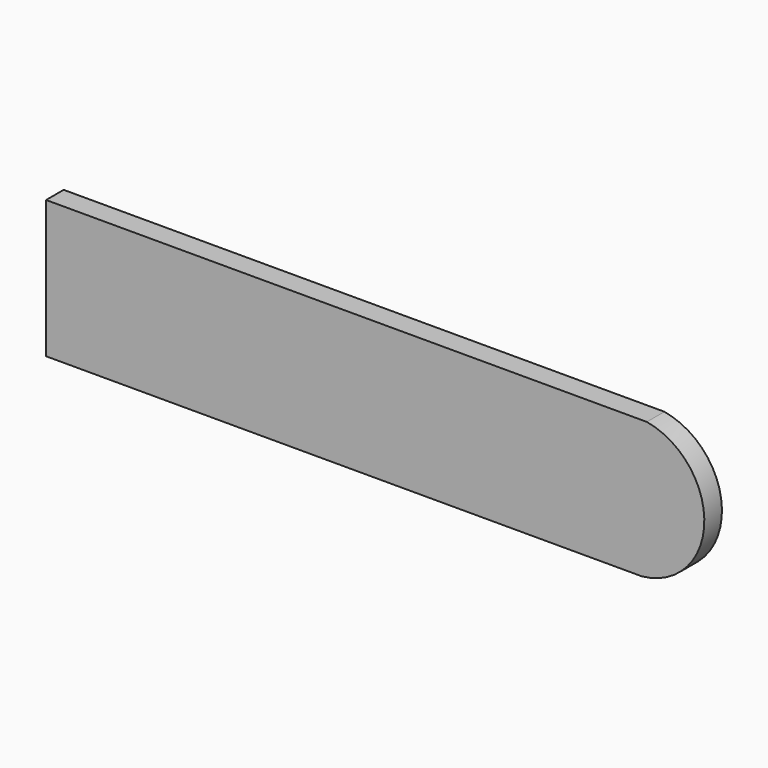
from build123d import *

# Parameters (mm, degrees)
F0_W     = 120
F0_H     = 25
F1_DEPTH = 4
F3_DEPTH = 4.001


# Not quite as in the source:
# - a feature of the source that left no trace in its solid (it failed there, or was rolled back) is left out


with BuildPart() as f1:
    # F0 (on Front) → F1 (new body)
    with BuildSketch(Plane.XZ):
        with Locations((43.1125537308, 7.697368972)):
            Rectangle(F0_W, F0_H)
    extrude(amount=F1_DEPTH)

    # F2 (on face) → F3 (cut, through all)
    with BuildSketch(Plane.XZ.offset(4)):
        with BuildLine():
            ThreePointArc((92.2726206475, 20.197368972), (102.716373437, 7.3105662294), (91.3844667368, -4.802631028))
            Line((91.3844667368, -4.802631028), (103.1125537308, -4.802631028))
            Line((103.1125537308, -4.802631028), (103.1125537308, 20.197368972))
            Line((103.1125537308, 20.197368972), (92.2726206475, 20.197368972))
        make_face()
    extrude(amount=-F3_DEPTH, mode=Mode.SUBTRACT)


solid = f1.part
